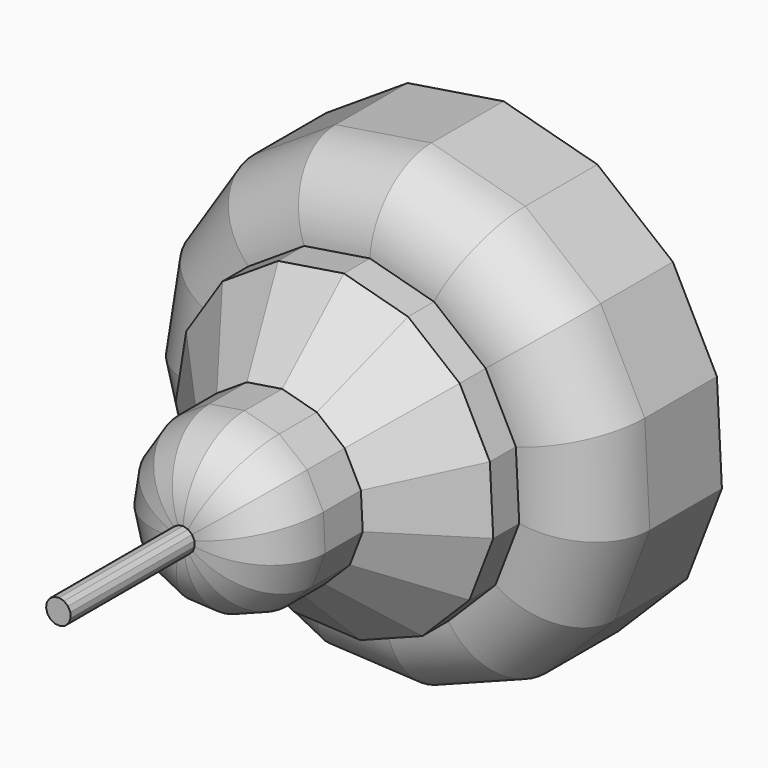
from build123d import *

# Parameters (mm, degrees)
F1_DEPTH = 11.43
F2_R     = 5.08
F3_DEPTH = 2.286
F4_DEPTH = 5.08
F5_SIZE  = 5.08
F6_DEPTH = 8.382
F7_R     = 5.08
F8_DEPTH = 10.922


with BuildPart() as f1:
    # F0 (on Front) → F1 (new body)
    with BuildSketch(Plane.XZ):
        Polygon((-5.8849686034, 15.3612454542), (-11.6241677455, 11.6395636341), (-15.3534426822, 5.9052955195), (-16.4279678975, -0.8500518383), (-14.6619482199, -7.4584175109), (-10.3607444954, -12.7771550382), (-4.2680739233, -15.8866063825), (2.5625854044, -16.2491191581), (8.9501504353, -13.8020116126), (13.7901531464, -8.968410872), (16.2457130989, -2.5840904161), (15.8922416689, 4.2470427484), (12.7908572779, 10.3438236386), (7.4778174622, 14.652063451), (0.8717950735, 16.4268283828), align=None)
    extrude(amount=F1_DEPTH)

    # F2
    f2_edges = [f1.edges().sort_by_distance(p)[0] for p in [
        (-2.506587, -11.43, 15.894037),
        (-8.754568, -11.43, 13.500405),
        (-13.488805, -11.43, 8.77243),
        (-15.890705, -11.43, 2.527622),
        (-15.544958, -11.43, -4.154235),
        (-12.511346, -11.43, -10.117786),
        (-7.314409, -11.43, -14.331881),
        (-0.852744, -11.43, -16.067863),
        (5.756368, -11.43, -15.025565),
        (11.370152, -11.43, -11.385211),
        (15.017933, -11.43, -5.776251),
        (16.068977, -11.43, 0.831476),
        (14.341549, -11.43, 7.295433),
        (10.134337, -11.43, 12.497944),
        (4.174806, -11.43, 15.539446),
    ]]
    fillet(f2_edges, radius=F2_R)

    # F3 (add): a face of the model
    f3_faces = [f1.faces().sort_by_distance(p)[0] for p in [
        (0, -11.43, 0),
    ]]
    extrude(f3_faces, amount=F3_DEPTH)

    # F4 (add): a face of the model
    f4_faces = [f1.faces().sort_by_distance(p)[0] for p in [
        (0, -13.716, 0),
    ]]
    extrude(f4_faces, amount=F4_DEPTH)

    # F5
    f5_edges = [f1.edges().sort_by_distance(p)[0] for p in [
        (-5.990622, -18.796, 9.238128),
        (-1.71522, -18.796, 10.876055),
        (2.856758, -18.796, 10.633414),
        (6.934778, -18.796, 8.552159),
        (9.813711, -18.796, 4.992157),
        (10.995765, -18.796, 0.568967),
        (10.27655, -18.796, -3.952603),
        (7.780427, -18.796, -7.790732),
        (3.938998, -18.796, -10.281773),
        (-0.58352, -18.796, -10.995002),
        (-5.005142, -18.796, -9.807095),
        (-8.56133, -18.796, -6.923452),
        (-10.637186, -18.796, -2.842682),
        (-10.873776, -18.796, 1.729614),
        (-9.230191, -18.796, 6.002844),
    ]]
    chamfer(f5_edges, length=F5_SIZE)

    # F6 (add): a face of the model
    f6_faces = [f1.faces().sort_by_distance(p)[0] for p in [
        (0, -18.796, 0),
    ]]
    extrude(f6_faces, amount=F6_DEPTH)

    # F7
    f7_edges = [f1.edges().sort_by_distance(p)[0] for p in [
        (-3.226676, -27.178, 4.975851),
        (-0.923854, -27.178, 5.858074),
        (-4.971576, -27.178, 3.233259),
        (1.538711, -27.178, 5.727382),
        (-5.856846, -27.178, 0.931607),
        (3.735218, -27.178, 4.606374),
        (-5.729414, -27.178, -1.531129),
        (5.285873, -27.178, 2.688882),
        (-4.611314, -27.178, -3.729118),
        (5.922552, -27.178, 0.306458),
        (-2.695876, -27.178, -5.282309),
        (5.535168, -27.178, -2.128956),
        (-0.314296, -27.178, -5.922141),
        (4.190703, -27.178, -4.196253),
        (2.121628, -27.178, -5.537981),
    ]]
    fillet(f7_edges, radius=F7_R)

    # F8 (add): a face of the model
    f8_faces = [f1.faces().sort_by_distance(p)[0] for p in [
        (0, -27.178, 0),
    ]]
    extrude(f8_faces, amount=F8_DEPTH)


solid = f1.part
